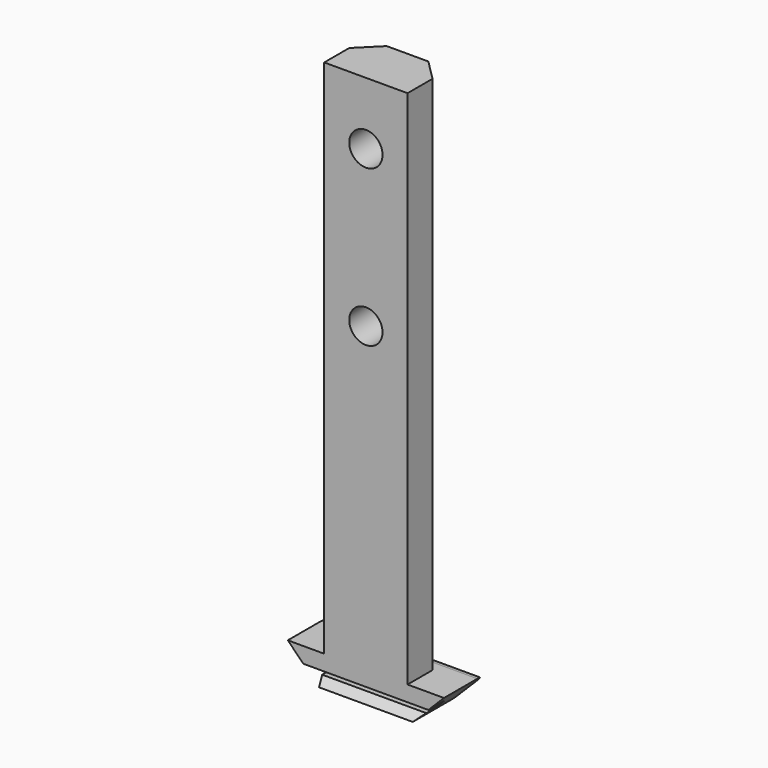
from build123d import *

# Parameters (mm, degrees)
F0_W           = 8
F0_H           = 50
F1_DEPTH       = 2.5
F2_W           = 15
F2_H           = 1
F2_W_2         = 0.5
F3_DEPTH       = 2
F4_SIZE        = 2.99999
F5_SIZE        = 2
F6_SIZE2       = 0.49999
F6_SIZE        = 0.99999
F7_R           = 1
F9_D           = 3.2
F9_CSINK_D     = 4
F9_CSINK_ANGLE = 82


# Not quite as in the source:
# - a fillet or chamfer is up to 0.001 mm smaller than in the source, because OpenCascade refuses the exact size


with BuildPart() as f1:
    # F0 (on Front) → F1 (new body, symmetric)
    with BuildSketch(Plane.XZ):
        Rectangle(F0_W, F0_H)
        Polygon((7.5, -25), (4, -25), (-4, -25), (-7.5, -25), (-7.5, -28), (7.5, -28), align=None)
    extrude(amount=F1_DEPTH, both=True)

    # F2 (on face) → F3 (cut)
    with BuildSketch(Plane.XZ.offset(2.5)):
        with Locations((0, -27)):
            Rectangle(F2_W, F2_H)
        with Locations((-7.75, -27)):
            Rectangle(F2_W_2, F2_H)
        with Locations((7.75, -27)):
            Rectangle(F2_W_2, F2_H)
    extrude(amount=-F3_DEPTH, mode=Mode.SUBTRACT)

    # F4 (size 3 in the source; OpenCascade refuses exactly that, so slightly less here)
    f4_edges = [f1.edges().sort_by_distance(p)[0] for p in [
        (-7.5, 0, -28),
        (7.5, 0, -28),
    ]]
    chamfer(f4_edges, length=F4_SIZE)

    # F5
    f5_edges = [f1.edges().sort_by_distance(p)[0] for p in [
        (-4, 2.5, 0),
        (4, 2.5, 0),
    ]]
    chamfer(f5_edges, length=F5_SIZE)

    # F6 (size 1 and 0.5 in the source; OpenCascade refuses exactly that, so slightly less here)
    f6_edges = [f1.edges().sort_by_distance(p)[0] for p in [
        (0, -2.5, -27.5),
    ]]
    f6_side = f1.faces().sort_by_distance((0, -1.5, -27.5))[0]
    chamfer(f6_edges, length=F6_SIZE, length2=F6_SIZE2, reference=f6_side)

    # F7
    f7_edges = [f1.edges().sort_by_distance(p)[0] for p in [
        (-5.75, 2.5, -25),
        (5.75, 2.5, -25),
    ]]
    fillet(f7_edges, radius=F7_R)

    # F9 (through all)
    with Locations(Plane(origin=(0, 2.5, 0), x_dir=(-1, 0, 0), z_dir=(0, 1, 0))):
        with Locations((0, 19), (0, 4)):
            CounterSinkHole(F9_D / 2, F9_CSINK_D / 2, counter_sink_angle=F9_CSINK_ANGLE)


solid = f1.part
